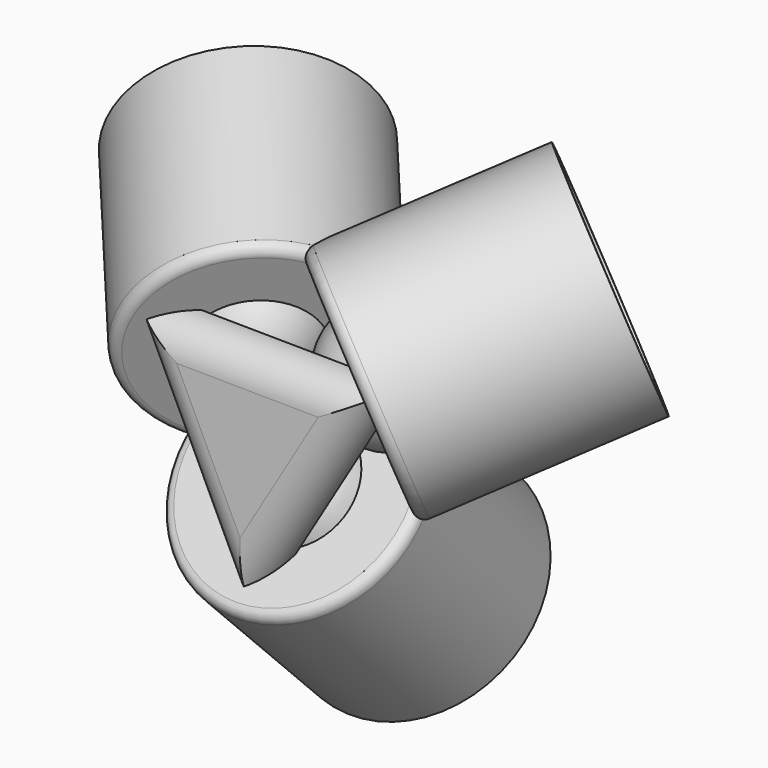
from build123d import *

# Parameters (mm, degrees)
F2_R      = 1.5
F4_COUNT  = 3
F6_ANGLE  = 45
F7_ANGLE  = -45
F8_ANGLE  = 45
F9_DEPTH  = 27.79057
F10_DEPTH = 27.79057
F11_DEPTH = 27.79057
F17_DEPTH = 5
F18_R     = 4.99999


# Not quite as in the source:
# - a fillet or chamfer is up to 0.001 mm smaller than in the source, because OpenCascade refuses the exact size


with BuildPart() as f1:
    # F0 (on Front) → F1 (revolve)
    with BuildSketch(Plane.XZ):
        with BuildLine():
            Line((9.3661535876, 12.8847169811), (13.39, 12.8847169811))
            Line((13.39, 12.8847169811), (13.39, -8.5594598204))
            Line((13.39, -8.5594598204), (15.39, -14.9058490566))
            Line((15.39, -14.9058490566), (17.39, -14.9058490566))
            Line((17.39, -14.9058490566), (17.39, 16.8847169811))
            Line((17.39, 16.8847169811), (8.4690514833, 16.8847169811))
            ThreePointArc((8.4690514833, 16.8847169811), (5.0129940493, 20.7963997154), (0, 22.2508705687))
            Line((0, 22.2508705687), (0, 19.6122665526))
            ThreePointArc((0, 19.6122665526), (4.7570959228, 17.6418129039), (6.7275495715, 12.8847169811))
            Line((6.7275495715, 12.8847169811), (9.3661535876, 12.8847169811))
        make_face()
    revolve(axis=Axis((0, 0, 12.7783455608), (0, 0, 1)))

    # F2
    f2_edges = [f1.edges().sort_by_distance(p)[0] for p in [
        (-17.39, 0, 16.884717),
    ]]
    fillet(f2_edges, radius=F2_R)


with BuildPart() as f4_1:
    # F4: instance of F1
    add(f1.part.rotate(Axis((0, -13.616835, 26), (0, 1, 0)), 1 * 360 / F4_COUNT))


with BuildPart() as f4_2:
    # F4: instance of F1
    add(f1.part.rotate(Axis((0, -13.616835, 26), (0, 1, 0)), 2 * 360 / F4_COUNT))


with BuildPart() as f1_1:
    add(f1.part)

    # F0 (on Front) → F5 (revolve, cut)
    with BuildSketch(Plane.XZ):
        Polygon((13.39, -8.5594598204), (13.39, 12.8847169811), (9.3661535876, 12.8847169811), (6.7275495715, 12.8847169811), (0, 12.8847169811), (0, -10.1359616965), (13.39, -10.1359616965), align=None)
    revolve(axis=Axis((0, 0, 1.3743776423), (0, 0, 1)), mode=Mode.SUBTRACT)


with BuildPart() as f1_2:
    # F6: moved
    add(f1_1.part.rotate(Axis((-3.022489244, 0, 14.9058490566), (1, 0, 0)), F6_ANGLE))


with BuildPart() as f4_1_1:
    # F7: moved
    add(f4_1.part.rotate(Axis((-7.7055660377, 0, 28.2522809351), (0.5, 0, 0.8660254038)), F7_ANGLE))


with BuildPart() as f4_2_1:
    # F8: moved
    add(f4_2.part.rotate(Axis((7.7055660377, 0, 28.2522809351), (-0.5, 0, 0.8660254038)), F8_ANGLE))


with BuildPart() as f9_tool:
    # F9 (cut): a face of the model
    f9_faces = [f1_2.part.faces().sort_by_distance(p)[0] for p in [
        (-13.011273608, 1.4291561963, 13.4766928604),
    ]]
    extrude(f9_faces, amount=F9_DEPTH)


with BuildPart() as f4_1_2:
    add(f4_1_1.part)

    # F9: cut by f9_tool
    add(f9_tool.part, mode=Mode.SUBTRACT)


with BuildPart() as f4_2_2:
    add(f4_2_1.part)

    # F9: cut by f9_tool
    add(f9_tool.part, mode=Mode.SUBTRACT)


with BuildPart() as f10_tool:
    # F10 (cut): a face of the model
    f10_faces = [f4_2_2.part.faces().sort_by_distance(p)[0] for p in [
        (16.5154045129, 3.7589277557, 20.5110486011),
    ]]
    extrude(f10_faces, amount=F10_DEPTH)


with BuildPart() as f1_3:
    add(f1_2.part)

    # F10: cut by f10_tool
    add(f10_tool.part, mode=Mode.SUBTRACT)


with BuildPart() as f4_1_3:
    add(f4_1_2.part)

    # F10: cut by f10_tool
    add(f10_tool.part, mode=Mode.SUBTRACT)


with BuildPart() as f11_tool:
    # F11 (cut): a face of the model
    f11_faces = [f4_1_3.part.faces().sort_by_distance(p)[0] for p in [
        (-7.192664292, 11.3085047439, 21.5593543531),
    ]]
    extrude(f11_faces, amount=F11_DEPTH)


with BuildPart() as f1_4:
    add(f1_3.part)

    # F11: cut by f11_tool
    add(f11_tool.part, mode=Mode.SUBTRACT)


with BuildPart() as f4_2_3:
    add(f4_2_2.part)

    # F11: cut by f11_tool
    add(f11_tool.part, mode=Mode.SUBTRACT)


with BuildPart() as f17:
    # F16 (on 3pt) → F17 (new body)
    with BuildSketch(Plane(origin=(0, -12.7779963754, 0.8841844204), x_dir=(1, 0, 0), z_dir=(0, -0.9976145296, 0.0690307931))):
        Polygon((19.185565412, 36.1157096922), (-18.9822055399, 36.4915132523), (0, 2.1474533714), align=None)
    extrude(amount=-F17_DEPTH)

    # F18 (radius 5 in the source; OpenCascade refuses exactly that, so slightly less here)
    f18_edges = [f17.edges().sort_by_distance(p)[0] for p in [
        (9.592783, -11.457328, 19.970128),
        (0.10168, -10.271929, 37.101195),
        (-9.491103, -11.444357, 20.157582),
    ]]
    fillet(f18_edges, radius=F18_R)


solid = Compound([f4_1_3.part, f1_4.part, f4_2_3.part, f17.part])
